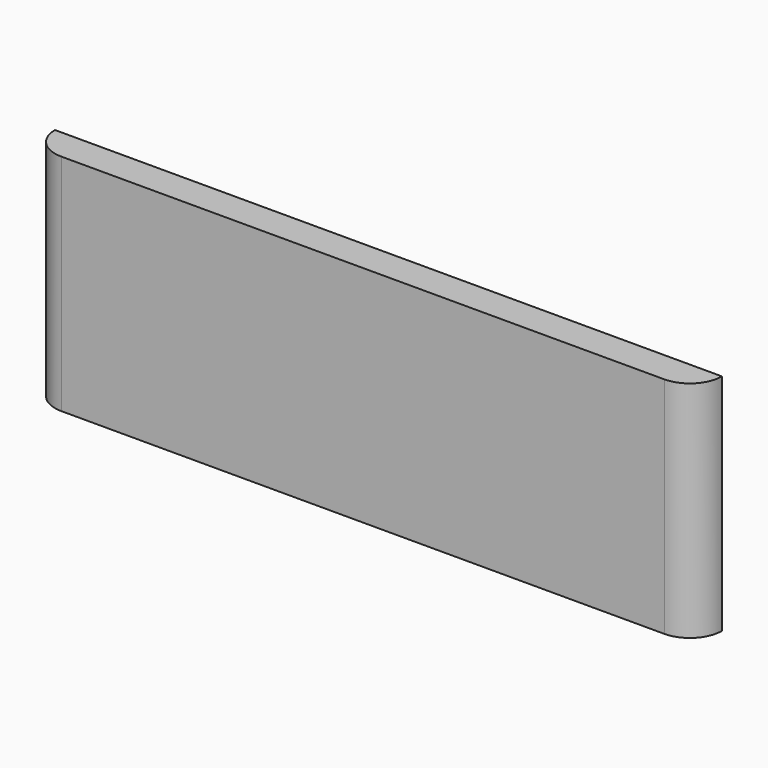
from build123d import *

# Parameters (mm, degrees)
F0_W     = 396.875
F0_H     = 133.35
F1_DEPTH = 19.05
F2_R     = 19.04999


# Not quite as in the source:
# - a fillet or chamfer is up to 0.001 mm smaller than in the source, because OpenCascade refuses the exact size


with BuildPart() as f1:
    # F0 (on Front) → F1 (new body)
    with BuildSketch(Plane.XZ):
        Rectangle(F0_W, F0_H)
    extrude(amount=F1_DEPTH)

    # F2 (radius 19.05 in the source; OpenCascade refuses exactly that, so slightly less here)
    f2_edges = [f1.edges().sort_by_distance(p)[0] for p in [
        (-198.4375, -19.05, 0),
        (198.4375, -19.05, 0),
    ]]
    fillet(f2_edges, radius=F2_R)


solid = f1.part
